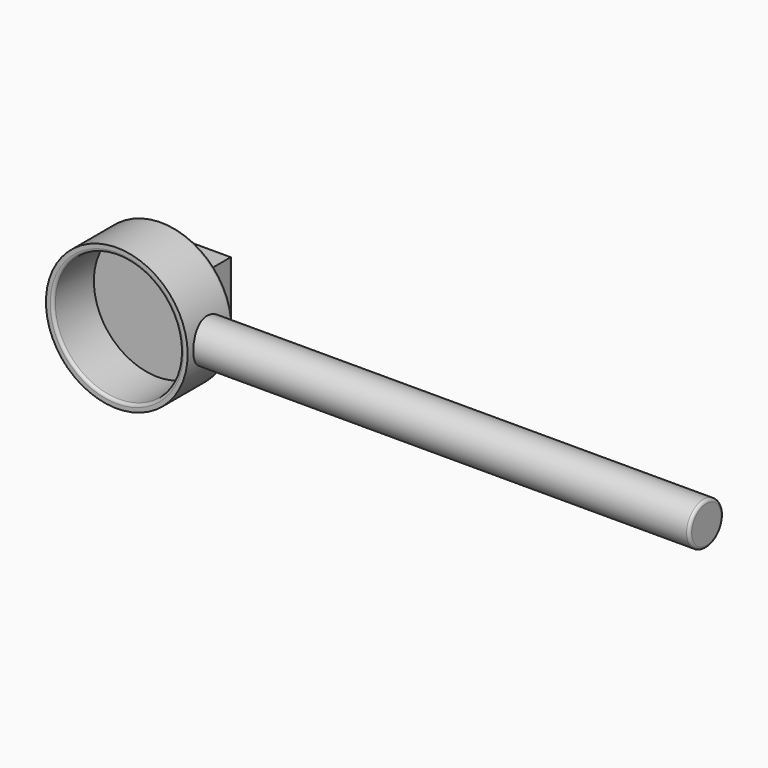
from build123d import *

# Parameters (mm, degrees)
F0_R     = 12.5
F1_DEPTH = 10
F2_R     = 11.25
F3_DEPTH = 9
F4_W     = 9.525
F4_H     = 9.525
F5_DEPTH = 9.525
F7_START = 11.25
F6_R     = 3.75
F7_DEPTH = 88.75
F8_R     = 1.25
F9_DEPTH = 1
F10_R    = 0.99999
F11_R    = 0.5
F11_2_R  = 0.5


# Not quite as in the source:
# - a fillet or chamfer is up to 0.001 mm smaller than in the source, because OpenCascade refuses the exact size


with BuildPart() as f1:
    # F0 (on Front) → F1 (new body)
    with BuildSketch(Plane.XZ):
        Circle(F0_R)
    extrude(amount=F1_DEPTH)

    # F2 (on face) → F3 (cut)
    with BuildSketch(Plane.XZ.offset(10)):
        Circle(F2_R)
    extrude(amount=-F3_DEPTH, mode=Mode.SUBTRACT)

    # F4 (on face) → F5 (join)
    with BuildSketch(Plane(origin=(0, 0, 0), x_dir=(-1, 0, 0), z_dir=(0, 1, 0))):
        Rectangle(F4_W, F4_H)
    extrude(amount=F5_DEPTH)

    # F8 (on face) → F9 (join)
    with BuildSketch(Plane(origin=(0, 0, -4.7625), x_dir=(1, 0, 0), z_dir=(0, 0, -1))):
        with Locations((0, -4.7625)):
            Circle(F8_R)
    extrude(amount=F9_DEPTH)

    # F10 (radius 1 in the source; OpenCascade refuses exactly that, so slightly less here)
    f10_edges = [f1.edges().sort_by_distance(p)[0] for p in [
        (-1.25, 4.7625, -5.7625),
    ]]
    fillet(f10_edges, radius=F10_R)

    # F11
    f11_edges = [f1.edges().sort_by_distance(p)[0] for p in [
        (0, 9.525, -4.7625),
        (-4.7625, 9.525, 0),
        (0, 9.525, 4.7625),
        (4.7625, 9.525, 0),
        (-11.25, -10, 0),
        (-12.5, 0, 0),
    ]]
    fillet(f11_edges, radius=F11_R)


with BuildPart() as f7:
    # F6 (on Right) → F7 (new body)
    with BuildSketch(Plane.YZ.offset(F7_START)):
        with Locations((-5, 0)):
            Circle(F6_R)
    extrude(amount=F7_DEPTH)

    # F11#2
    f11_2_edges = [f7.edges().sort_by_distance(p)[0] for p in [
        (55.625, -1.25, 0),
        (11.25, -8.75, 0),
        (100, -8.75, 0),
    ]]
    fillet(f11_2_edges, radius=F11_2_R)


solid = Compound([f1.part, f7.part])
